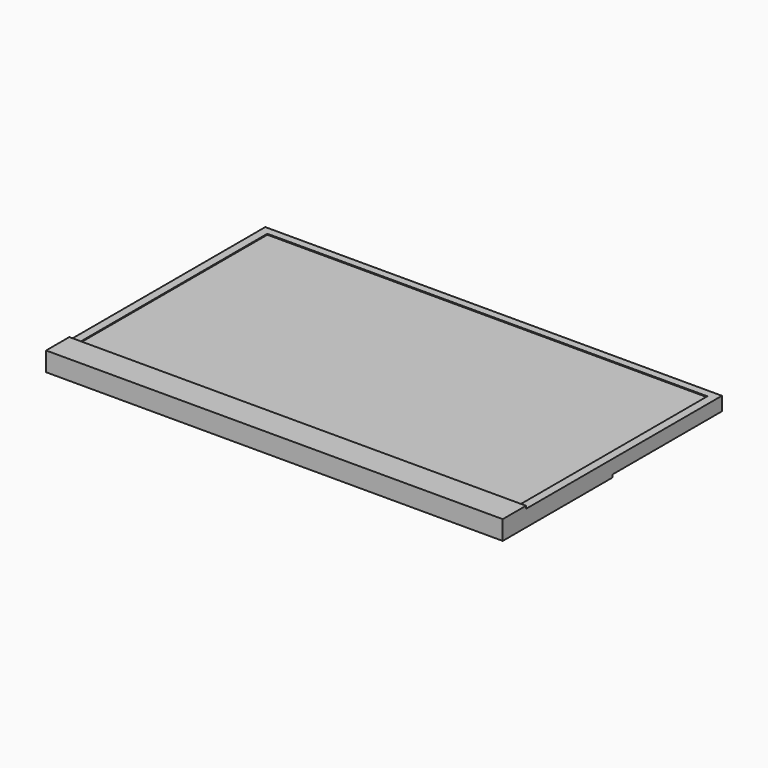
from build123d import *

# Parameters (mm, degrees)
F0_W      = 500
F0_H      = 300
F1_DEPTH  = 15
F2_W      = 481.8210515528
F2_H      = 257.048019406
F3_DEPTH  = 1
F4_W      = 500
F4_H      = 150
F5_DEPTH  = 3
F6_W      = 127
F6_H      = 68
F7_DEPTH  = 5
F8_SIZE2  = 2.886741
F8_SIZE   = 4.99999
F9_W      = 102.6
F9_H      = 44
F10_DEPTH = 10
F11_W     = 167
F11_H     = 82
F12_DEPTH = 20
F13_R     = 2.1
F14_DEPTH = 20
F15_R     = 3.85
F16_DEPTH = 12.5
F17_W     = 17.7404675633
F17_H     = 6.0484888963
F17_W_2   = 11.7162363604
F17_H_2   = 5.917977076
F17_R     = 3.0117076701
F17_R_2   = 3.5627139526
F18_DEPTH = 5
F19_W     = 500
F19_H     = 31.8
F20_DEPTH = 3
F21_R     = 1.9
F21_W     = 40.1
F21_H     = 6.3
F22_DEPTH = 1
F23_W     = 119.3
F23_H     = 28.2
F24_DEPTH = 5.8
F25_W     = 23
F25_H     = 23
F26_DEPTH = 15
F28_DEPTH = 8.6
F29_R     = 2
F30_DEPTH = 1.5
F31_R     = 8
F32_DEPTH = 1


# Not quite as in the source:
# - a fillet or chamfer is up to 0.001 mm smaller than in the source, because OpenCascade refuses the exact size
# - a pattern or mirror of a feature is missing from the dataset's text; its kind, count and spacing are read off the source's solid


with BuildPart() as f1:
    # F0 (on Top) → F1 (new body)
    with BuildSketch(Plane.XY):
        Rectangle(F0_W, F0_H)
    extrude(amount=F1_DEPTH)

    # F2 (on face) → F3 (cut)
    with BuildSketch(Plane.XY.offset(15)):
        with Locations((0, 12.9358926788)):
            Rectangle(F2_W, F2_H)
    extrude(amount=-F3_DEPTH, mode=Mode.SUBTRACT)

    # F4 (on face) → F5 (join)
    with BuildSketch(Plane(origin=(0, 0, 0), x_dir=(1, 0, 0), z_dir=(0, 0, -1))):
        with Locations((0, 75)):
            Rectangle(F4_W, F4_H)
    extrude(amount=F5_DEPTH)

    # F6 (on face) → F7 (join)
    with BuildSketch(Plane(origin=(0, 0, -3), x_dir=(1, 0, 0), z_dir=(0, 0, -1))):
        with Locations((0, 44)):
            Rectangle(F6_W, F6_H)
    extrude(amount=F7_DEPTH)

    # F8 (size 5 and 2.8867513459 in the source; OpenCascade refuses exactly that, so slightly less here)
    f8_edges = [f1.edges().sort_by_distance(p)[0] for p in [
        (0, -78, -8),
        (-63.5, -44, -8),
        (0, -10, -8),
        (63.5, -44, -8),
    ]]
    chamfer(f8_edges, length=F8_SIZE, length2=F8_SIZE2)

    # F9 (on face) → F10 (cut)
    with BuildSketch(Plane(origin=(0, 0, -8), x_dir=(1, 0, 0), z_dir=(0, 0, -1))):
        with Locations((0, 44)):
            Rectangle(F9_W, F9_H)
    extrude(amount=-F10_DEPTH, mode=Mode.SUBTRACT)

    # F19 (on face) → F20 (join)
    with BuildSketch(Plane.XY.offset(15)):
        with Locations((0, -134.1)):
            Rectangle(F19_W, F19_H)
    extrude(amount=F20_DEPTH)

    # F21 (on face) → F22 (cut)
    with BuildSketch(Plane(origin=(0, 0, 2), x_dir=(1, 0, 0), z_dir=(0, 0, -1))):
        with Locations((-16.15, 43)):
            Circle(F21_R)
        with Locations((-16.15, 54)):
            Circle(F21_R)
        with Locations((16.15, 54)):
            Circle(F21_R)
        with Locations((16.15, 43)):
            Circle(F21_R)
        with Locations((0, 35.95)):
            Rectangle(F21_W, F21_H)
    extrude(amount=-F22_DEPTH, mode=Mode.SUBTRACT)


with BuildPart() as f12:
    # F11 (on face) → F12 (new body)
    with BuildSketch(Plane(origin=(0, 0, 0), x_dir=(1, 0, 0), z_dir=(0, 0, -1))):
        with Locations((0, -51)):
            Rectangle(F11_W, F11_H)
    extrude(amount=F12_DEPTH)

    # F13 (on face) → F14 (cut, through all)
    with BuildSketch(Plane(origin=(0, 0, -20), x_dir=(1, 0, 0), z_dir=(0, 0, -1))):
        with Locations((64.9, -85.6)):
            Circle(F13_R)
        with Locations((78.3, -15.1)):
            Circle(F13_R)
        with Locations((-76.9, -85.6)):
            Circle(F13_R)
        with Locations((-76.9, -15.1)):
            Circle(F13_R)
    extrude(amount=-F14_DEPTH, mode=Mode.SUBTRACT)

    # F15 (on face) → F16 (cut)
    with BuildSketch(Plane.XY):
        with Locations((-76.9, 15.1)):
            Circle(F15_R)
        with Locations((-76.9, 85.6)):
            Circle(F15_R)
        with Locations((64.9, 85.6)):
            Circle(F15_R)
        with Locations((78.3, 15.1)):
            Circle(F15_R)
    extrude(amount=-F16_DEPTH, mode=Mode.SUBTRACT)

    # F17 (on face) → F18 (join)
    with BuildSketch(Plane(origin=(0, 92, 0), x_dir=(-1, 0, 0), z_dir=(0, 1, 0))):
        with Locations((-17.5635432824, -9.4999487046)):
            Rectangle(F17_W, F17_H)
        with Locations((16.5168526582, -10.5239257682)):
            Rectangle(F17_W_2, F17_H_2)
        with Locations((44.8921956122, -10.3334598243)):
            Circle(F17_R)
        with Locations((60.8012191951, -10.3334598243)):
            Circle(F17_R_2)
    extrude(amount=F18_DEPTH)


with BuildPart() as f24:
    # F23 (on face) → F24 (new body)
    with BuildSketch(Plane(origin=(0, 0, 0), x_dir=(1, 0, 0), z_dir=(0, 0, -1))):
        with Locations((0, -116.1)):
            Rectangle(F23_W, F23_H)
    extrude(amount=F24_DEPTH)


with BuildPart() as f26:
    # F25 (on face) → F26 (new body)
    with BuildSketch(Plane(origin=(0, 0, 0), x_dir=(1, 0, 0), z_dir=(0, 0, -1))):
        with Locations((0, -151.7)):
            Rectangle(F25_W, F25_H)
    extrude(amount=F26_DEPTH)

    # F27 (on face) → F28 (join)
    with BuildSketch(Plane(origin=(-11.5, 0, 0), x_dir=(0, -1, 0), z_dir=(-1, 0, 0))):
        Polygon((-149.7414580757, -11.7), (-143.5, -1.5), (-145.2585419243, -1.5), (-151.5, -11.7), align=None)
    f28 = extrude(amount=F28_DEPTH)

    # F28_copies: F28 across plane
    add(f28.mirror(Plane(origin=(0, 0, 0), x_dir=(0, 0, 1), z_dir=(1, 0, 0))))

    # F29 (on face) → F30 (cut, through all)
    with BuildSketch(Plane(origin=(0, 103.7390315274, 63.4787074597), x_dir=(1, 0, 0), z_dir=(0, -0.8529793798, -0.5219446116))):
        with Locations((-15.8, -82.1575633804)):
            Circle(F29_R)
    f30 = extrude(amount=-F30_DEPTH, mode=Mode.SUBTRACT)

    # F30_copies: F30 across plane
    add(f30.mirror(Plane(origin=(0, 0, 0), x_dir=(0, 0, 1), z_dir=(1, 0, 0))), mode=Mode.SUBTRACT)

    # F31 (on face) → F32 (cut)
    with BuildSketch(Plane(origin=(0, 0, -15), x_dir=(1, 0, 0), z_dir=(0, 0, -1))):
        with Locations((0, -151.7)):
            Circle(F31_R)
    extrude(amount=-F32_DEPTH, mode=Mode.SUBTRACT)


solid = Compound([f1.part, f12.part, f24.part, f26.part])
